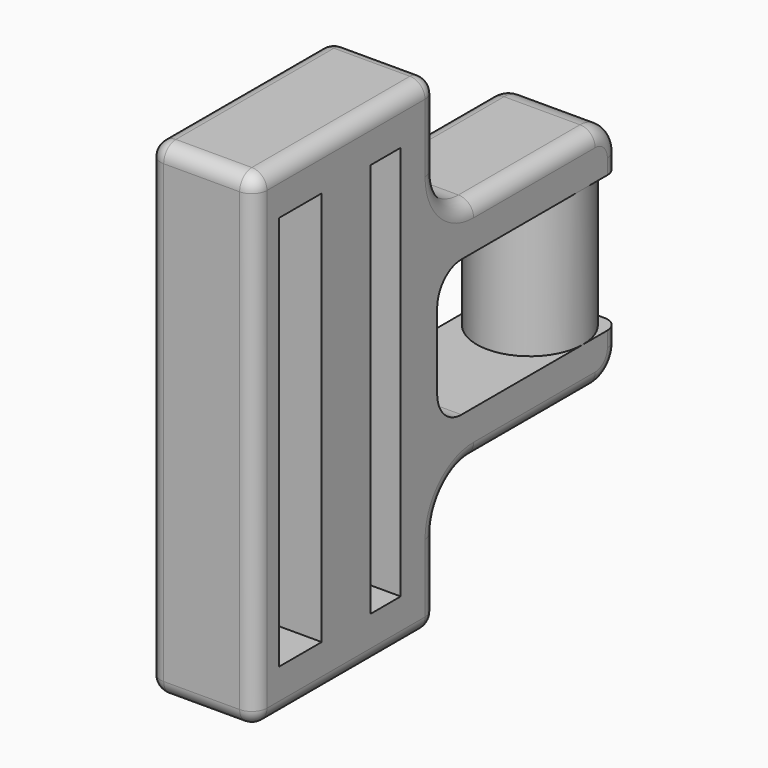
from build123d import *

# Parameters (mm, degrees)
F0_W      = 15
F0_H      = 3
F0_W_2    = 1.5
F0_H_2    = 26
F0_W_3    = 2.5
F1_DEPTH  = 3.5
F2_R      = 3.5
F3_DEPTH  = 9
F4_R      = 1
F5_R      = 3
F6_R      = 2
F7_R      = 1
F8_SIZE2  = 1.99999
F8_SIZE   = 6.99999
F9_W      = 4
F9_H      = 26
F10_DEPTH = 4


# Not quite as in the source:
# - a fillet or chamfer is up to 0.001 mm smaller than in the source, because OpenCascade refuses the exact size


with BuildPart() as f1:
    # F0 (on Right) → F1 (new body, symmetric)
    with BuildSketch(Plane.YZ):
        with Locations((-4.5, 6)):
            Rectangle(F0_W, F0_H)
        Polygon((-12, -4.5), (-12, 4.5), (-12, 7.5), (-12, 16), (-27, 16), (-27, -16), (-12, -16), (-12, -7.5), align=None)
        with Locations((-22.25, 0)):
            Rectangle(F0_W_2, F0_H_2, mode=Mode.SUBTRACT)
        with Locations((-16.25, 0)):
            Rectangle(F0_W_3, F0_H_2, mode=Mode.SUBTRACT)
        with Locations((-4.5, -6)):
            Rectangle(F0_W, F0_H)
    extrude(amount=F1_DEPTH, both=True)

    # F2 (on face) → F3 (join, through all)
    with BuildSketch(Plane.XY.offset(-4.5)):
        Circle(F2_R)
    extrude(amount=F3_DEPTH)

    # F4
    f4_edges = [f1.edges().sort_by_distance(p)[0] for p in [
        (0, -27, 16),
        (0, -12, 16),
        (0, -27, -16),
        (0, -12, -16),
    ]]
    fillet(f4_edges, radius=F4_R)

    # F5
    f5_edges = [f1.edges().sort_by_distance(p)[0] for p in [
        (0, -12, 7.5),
        (0, -12, -7.5),
    ]]
    fillet(f5_edges, radius=F5_R)

    # F6
    f6_edges = [f1.edges().sort_by_distance(p)[0] for p in [
        (0, 3, 7.5),
        (0, 3, -7.5),
        (0, -12, -4.5),
        (0, -12, 4.5),
    ]]
    fillet(f6_edges, radius=F6_R)

    # F7
    f7_edges = [f1.edges().sort_by_distance(p)[0] for p in [
        (-3.5, -4, -7.5),
        (-3.5, -4, 7.5),
        (3.5, 2.414214, 6.914214),
        (3.5, 2.414214, -6.914214),
    ]]
    fillet(f7_edges, radius=F7_R)

    # F8 (size 7 and 2 in the source; OpenCascade refuses exactly that, so slightly less here)
    f8_edges = [f1.edges().sort_by_distance(p)[0] for p in [
        (3.5, -23, 0),
    ]]
    f8_side = f1.faces().sort_by_distance((0, -23, 0))[0]
    chamfer(f8_edges, length=F8_SIZE, length2=F8_SIZE2, reference=f8_side)

    # F9 (on face) → F10 (cut)
    with BuildSketch(Plane(origin=(-3.5, 0, 0), x_dir=(0, -1, 0), z_dir=(-1, 0, 0))):
        with Locations((19.5, 0)):
            Rectangle(F9_W, F9_H)
    extrude(amount=-F10_DEPTH, mode=Mode.SUBTRACT)


solid = f1.part
